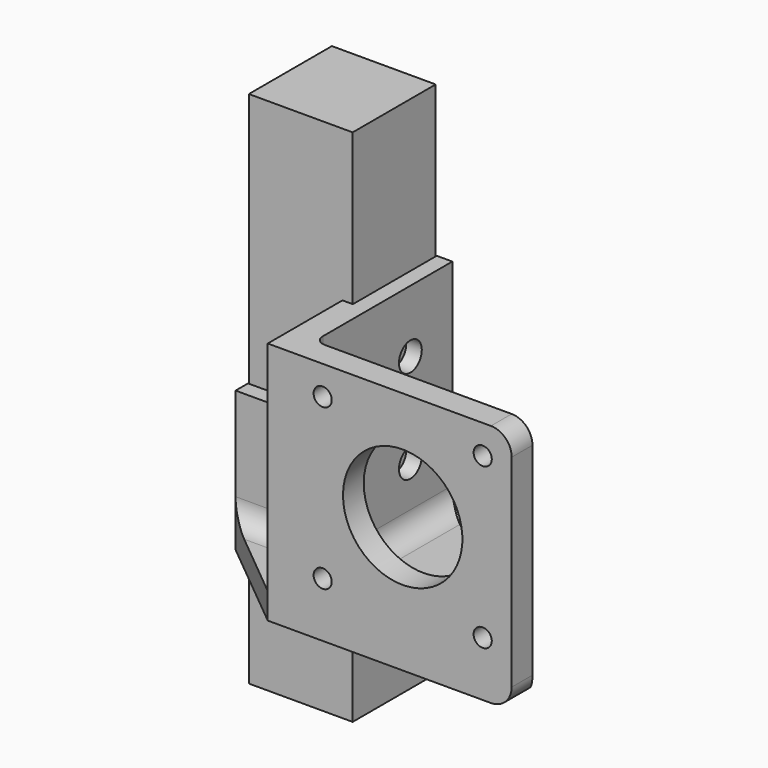
from build123d import *

# Parameters (mm, degrees)
F0_W      = 20
F0_H      = 20
F1_DEPTH  = 50
F3_DEPTH  = 21
F4_R      = 11.5
F4_R_2    = 1.75
F5_DEPTH  = 5.001
F7_DEPTH  = 5
F8_R      = 2.75
F9_DEPTH  = 3
F10_R     = 2.75
F11_DEPTH = 3
F12_R     = 4
F13_R     = 2
F14_W     = 18.2
F14_H     = 20
F14_R     = 2.75
F15_DEPTH = 25


# Not quite as in the source:
# - a feature names something its author has since deleted; it is built from what else it names


with BuildPart() as f1:
    # F0 (on Top) → F1 (new body, symmetric)
    with BuildSketch(Plane.XY):
        Rectangle(F0_W, F0_H)
    extrude(amount=F1_DEPTH, both=True)


with BuildPart() as f3:
    # F2 (on Top) → F3 (new body, symmetric)
    with BuildSketch(Plane.XY):
        Polygon((10.2, 10), (10.2, -10.2), (-10, -10.2), (-10, -13.2), (8.2, -13.2), (8.2, -28.2), (55.2, -28.2), (55.2, -23.2), (13.2, -23.2), (13.2, 10), align=None)
    extrude(amount=F3_DEPTH, both=True)

    # F4 (on face) → F5 (cut, through all)
    with BuildSketch(Plane(origin=(0, -23.2, 0), x_dir=(-1, 0, 0), z_dir=(0, 1, 0))):
        with Locations((-34.2, 0)):
            Circle(F4_R)
        with Locations((-49.6149278299, 15.4149278299)):
            Circle(F4_R_2)
        with Locations((-18.7850721701, 15.4149278299)):
            Circle(F4_R_2)
        with Locations((-18.7850721701, -15.4149278299)):
            Circle(F4_R_2)
        with Locations((-49.6149278299, -15.4149278299)):
            Circle(F4_R_2)
    extrude(amount=-F5_DEPTH, mode=Mode.SUBTRACT)

    # F6 (on face) → F7 (join)
    with BuildSketch(Plane(origin=(0, 0, -21), x_dir=(1, 0, 0), z_dir=(0, 0, -1))):
        Polygon((13.2, 23.2), (13.2, -10), (55.2, 23.2), align=None)
        Polygon((10.2, -10), (13.2, -10), (13.2, 23.2), (55.2, 23.2), (55.2, 28.2), (8.2, 28.2), (8.2, 13.2), (-10, 13.2), (-10, 10.2), (10.2, 10.2), align=None)
        Polygon((8.2, 13.2), (8.2, 28.2), (-10, 13.2), align=None)
    extrude(amount=F7_DEPTH)

    # F8 (on face) → F9 (cut, through all)
    with BuildSketch(Plane.XZ.offset(13.2)):
        with Locations((-0.9, 9)):
            Circle(F8_R)
        with Locations((-0.9, -9)):
            Circle(F8_R)
    extrude(amount=-F9_DEPTH, mode=Mode.SUBTRACT)

    # F10 (on face) → F11 (cut, through all)
    with BuildSketch(Plane.YZ.offset(13.2)):
        with Locations((-0.1, 9)):
            Circle(F10_R)
        with Locations((-0.1, -9)):
            Circle(F10_R)
    extrude(amount=-F11_DEPTH, mode=Mode.SUBTRACT)

    # F12
    f12_edges = [f3.edges().sort_by_distance(p)[0] for p in [
        (13.2, -6.6, -21),
        (-0.9, -13.2, -21),
        (55.2, -25.7, 21),
        (55.2, -25.7, -26),
    ]]
    fillet(f12_edges, radius=F12_R)

    # F13
    f13_edges = [f3.edges().sort_by_distance(p)[0] for p in [
        (36.2, -23.2, -21),
        (13.2, -23.2, 2),
        (14.371573, -23.2, -19.828427),
    ]]
    fillet(f13_edges, radius=F13_R)

    # F14 (on face) → F15 (cut)
    with BuildSketch(Plane.XZ.offset(13.2)):
        with Locations((-0.9, 11)):
            Rectangle(F14_W, F14_H)
        with Locations((-0.9, 9)):
            Circle(F14_R, mode=Mode.SUBTRACT)
    extrude(amount=-F15_DEPTH, mode=Mode.SUBTRACT)


solid = Compound([f1.part, f3.part])
